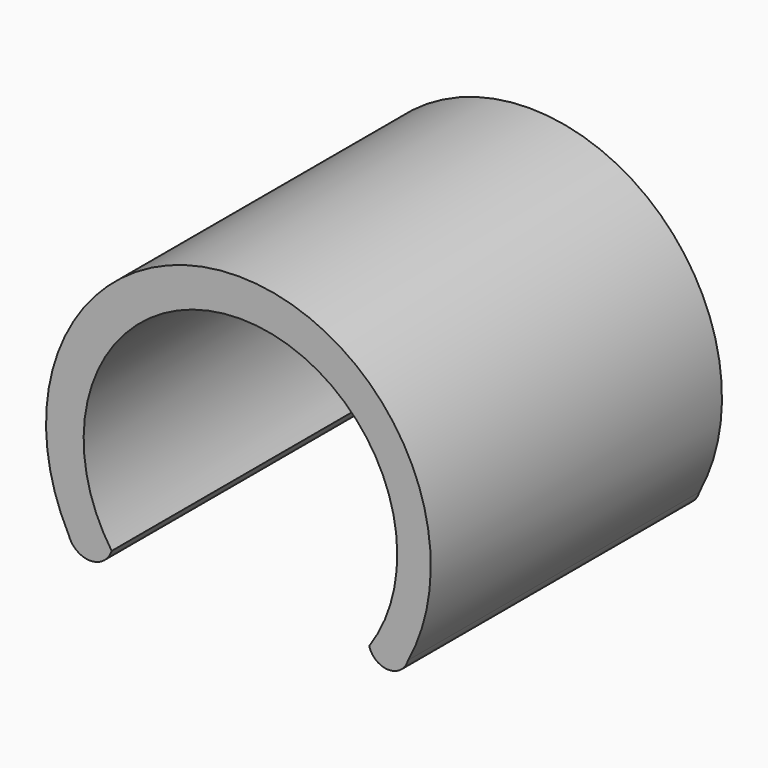
from build123d import *

# Parameters (mm, degrees)
F1_DEPTH = 50.8


# Not quite as in the source:
# - the program builds the solid bodies; features that only make, move or delete a surface that nothing else refers to are left out


with BuildPart() as f1:
    # F0 (on Front) → F1 (new body)
    with BuildSketch(Plane.XZ):
        with BuildLine():
            ThreePointArc((18.2554032654, 0), (20.9651887417, -2.0460110738), (23.674974218, 0))
            ThreePointArc((23.674974218, 0), (1.8626e-06, 39.5058318973), (-23.6749704927, 0))
            ThreePointArc((-23.6749704927, 0), (-20.6799441949, -2.1720430736), (-17.684917897, 0))
            ThreePointArc((-17.684917897, 0), (0.2852426842, 34.3693981049), (18.2554032654, 0))
        make_face()
    extrude(amount=F1_DEPTH)


solid = f1.part
